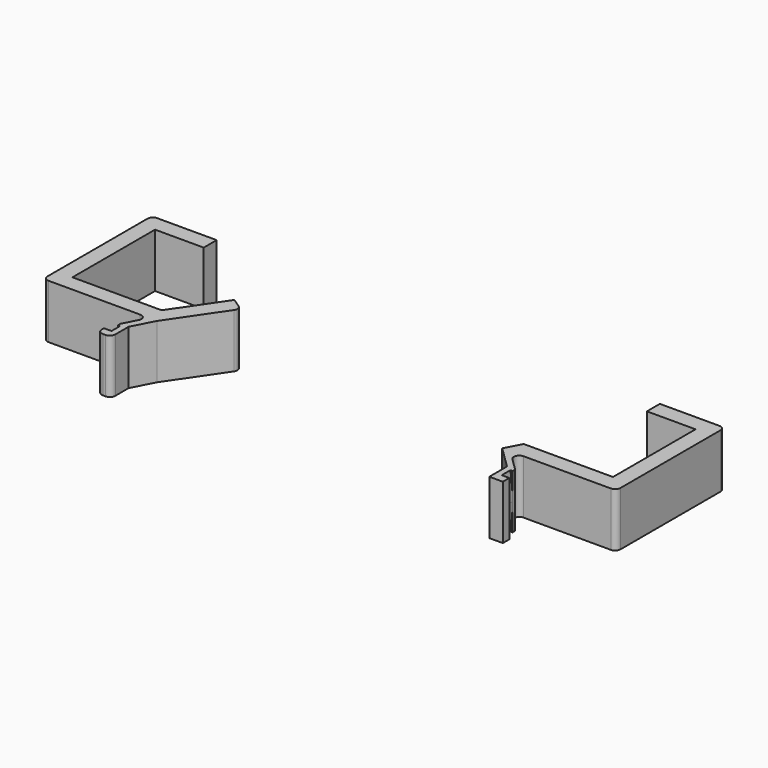
from build123d import *

# Parameters (mm, degrees)
F1_DEPTH = 5
F3_R     = 1
F3_2_R   = 1
F4_R     = 1
F4_2_R   = 1
F6_DEPTH = 2
F8_DEPTH = 2


# Not quite as in the source:
# - a feature names something its author has since deleted; it is built from what else it names


with BuildPart() as f1:
    # F0 (on Top) → F1 (new body, symmetric)
    with BuildSketch(Plane.XY):
        Polygon((103, 22.1), (91, 22.1), (91, 19.1), (100, 19.1), (100, 0), (83.5, 0), (81.9138380969, -3), (83.4138380969, -3), (103, -3), align=None)
        Polygon((87.5, -7), (83.4138380969, -3), (81.9138380969, -3), (86, -7), (86, -11.1), (88.5, -11.1), (88.5, -9.6), (87.5, -9.6), align=None)
    extrude(amount=F1_DEPTH, both=True)

    # F3
    f3_edges = [f1.edges().sort_by_distance(p)[0] for p in [
        (103, 22.1, 0),
        (103, -3, 0),
    ]]
    fillet(f3_edges, radius=F3_R)

    # F4
    f4_edges = [f1.edges().sort_by_distance(p)[0] for p in [
        (83.413838, -3, 0),
    ]]
    fillet(f4_edges, radius=F4_R)

    # F7 (on face) → F8 (cut)
    with BuildSketch(Plane(origin=(0, -9.6, 0), x_dir=(-1, 0, 0), z_dir=(0, 1, 0))):
        with BuildLine():
            ThreePointArc((-87.5, 0), (-87.39984051, 2.5079872408), (-87.1, 5))
            Line((-87.1, 5), (-87.5, 5))
            Line((-87.5, 5), (-87.5, 0))
        make_face()
        with BuildLine():
            ThreePointArc((-87.1, -5), (-87.39984051, -2.5079872408), (-87.5, 0))
            Line((-87.5, 0), (-87.5, -5))
            Line((-87.5, -5), (-87.1, -5))
        make_face()
    extrude(amount=F8_DEPTH, mode=Mode.SUBTRACT)


with BuildPart() as f1b:
    # F0 (on Top) → F1, piece 2 (new body, symmetric)
    with BuildSketch(Plane.XY):
        Polygon((16.5, 0), (0, 0), (0, 19.1), (9, 19.1), (9, 22.1), (-3, 22.1), (-3, -3), (16.5861619031, -3), (18.0861619031, -3), (25.1792582862, 7.4108350138), (22.7, 9.1), align=None)
        Polygon((16, -7), (18.0861619031, -3), (16.5861619031, -3), (14.5, -7), (14.5, -9.6), (13.5, -9.6), (13.5, -11.1), (16, -11.1), align=None)
    extrude(amount=F1_DEPTH, both=True)

    # F3#2
    f3_2_edges = [f1b.edges().sort_by_distance(p)[0] for p in [
        (13.5, -11.1, 0),
        (16, -11.1, 0),
        (25.179258, 7.410835, 0),
        (-3, -3, 0),
        (-3, 22.1, 0),
    ]]
    fillet(f3_2_edges, radius=F3_2_R)

    # F4#2
    f4_2_edges = [f1b.edges().sort_by_distance(p)[0] for p in [
        (16.586162, -3, 0),
    ]]
    fillet(f4_2_edges, radius=F4_2_R)

    # F5 (on face) → F6 (cut)
    with BuildSketch(Plane(origin=(0, -9.6, 0), x_dir=(-1, 0, 0), z_dir=(0, 1, 0))):
        with BuildLine():
            ThreePointArc((-14.9, 5), (-14.60015949, 2.5079872408), (-14.5, 0))
            Line((-14.5, 0), (-14.5, 5))
            Line((-14.5, 5), (-14.9, 5))
        make_face()
        with BuildLine():
            ThreePointArc((-14.5, 0), (-14.60015949, -2.5079872408), (-14.9, -5))
            Line((-14.9, -5), (-14.5, -5))
            Line((-14.5, -5), (-14.5, 0))
        make_face()
    extrude(amount=F6_DEPTH, mode=Mode.SUBTRACT)


solid = Compound([f1.part, f1b.part])
